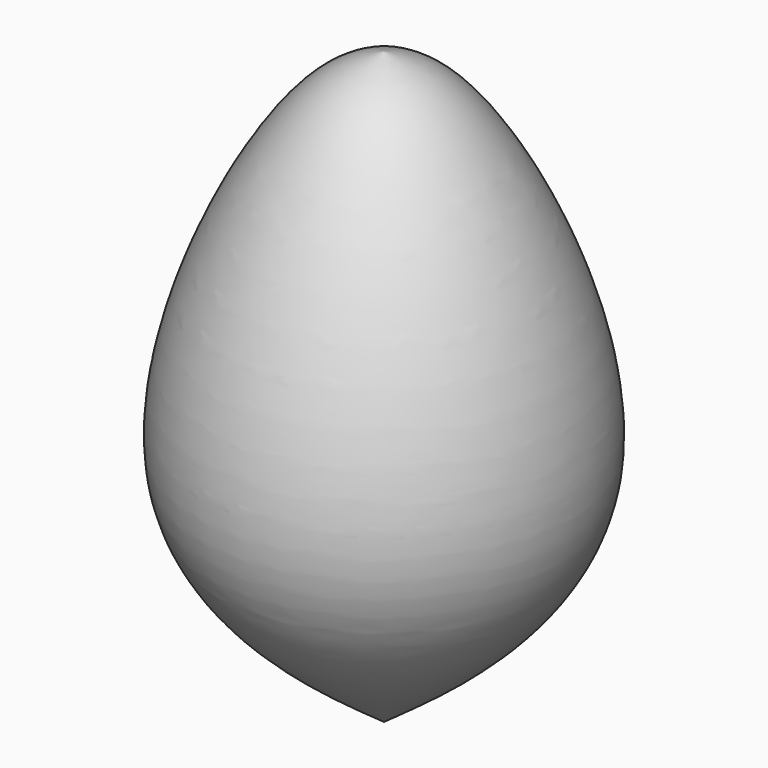
from build123d import *


with BuildPart() as f1:
    # F0 (on Front) → F1 (revolve)
    with BuildSketch(Plane.XZ):
        with BuildLine():
            Line((0, -11.3297364564), (0, 14.0702635436))
            add(Edge.make_bspline(
                [(0, -11.3297364564), (-3.7121922024, -8.6674044456), (-11.4420457382, -3.1236622617), (-3.9702111404, 12.8316439294), (-0.9963690021, 13.7594180632), (0, 14.0702635436)],
                knots=[0, 0, 0, 0, 0.3805740684, 0.7924648422, 1, 1, 1, 1], degree=3))
        make_face()
    revolve(axis=Axis((0, 0, 1.3702635436), (0, 0, -1)))


solid = f1.part
